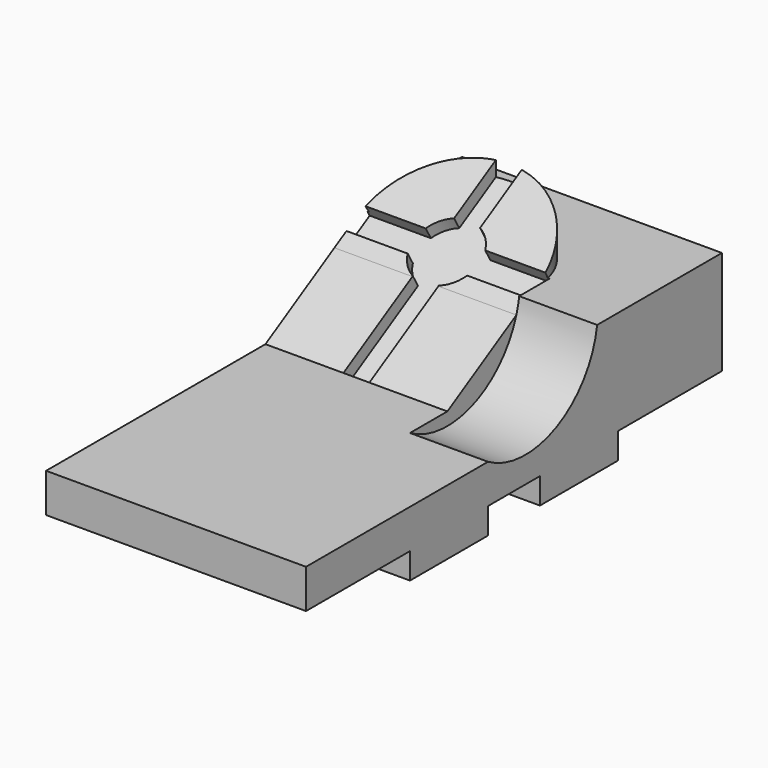
from build123d import *

# Parameters (mm, degrees)
F1_DEPTH  = 30
F0_W      = 37.5
F0_H      = 10
F2_DEPTH  = 100
F4_DEPTH  = 70
F5_W      = 20.9091625453
F5_H      = 25
F6_DEPTH  = 70
F7_DEPTH  = 70
F9_DEPTH  = 5
F12_DEPTH = 17.5


with BuildPart() as f1:
    # F0 (on Right) → F1 (new body)
    with BuildSketch(Plane.YZ):
        with BuildLine():
            Line((-100, 15), (-100, 0))
            Line((-100, 0), (-50, 0))
            Line((-50, 0), (-12.5, 0))
            Line((-12.5, 0), (12.5, 0))
            Line((12.5, 0), (50, 0))
            Line((50, 0), (100, 0))
            Line((100, 0), (100, 40))
            Line((100, 40), (40, 40))
            ThreePointArc((40, 40), (20.4711584909, 13.3855671691), (-12.5, 15))
            Line((-12.5, 15), (-100, 15))
        make_face()
    extrude(amount=-F1_DEPTH)

    # F0 (on Right) → F2 (join)
    with BuildSketch(Plane.YZ):
        with Locations((-31.25, -5)):
            Rectangle(F0_W, F0_H)
        with Locations((31.25, -5)):
            Rectangle(F0_W, F0_H)
    extrude(amount=-F2_DEPTH)

    # F3 (on face) → F4 (join)
    with BuildSketch(Plane(origin=(-30, 0, 0), x_dir=(0, -1, 0), z_dir=(-1, 0, 0))):
        with BuildLine():
            Line((12.5, 15), (-23.473678133, 15))
            ThreePointArc((-23.473678133, 15), (-34.5610974405, 25.633015883), (-40, 40))
            Line((-40, 40), (-100, 40))
            Line((-100, 40), (-100, 0))
            Line((-100, 0), (-50, 0))
            Line((-50, 0), (-12.5, 0))
            Line((-12.5, 0), (12.5, 0))
            Line((12.5, 0), (50, 0))
            Line((50, 0), (100, 0))
            Line((100, 0), (100, 15))
            Line((100, 15), (12.5, 15))
        make_face()
    extrude(amount=F4_DEPTH)

    # F5 (on face) → F6 (join)
    with BuildSketch(Plane(origin=(-100, 0, 0), x_dir=(0, -1, 0), z_dir=(-1, 0, 0))):
        with BuildLine():
            Line((-23.473678133, 15), (-5.478678133, 15))
            Line((-5.478678133, 15), (-38.6573392432, 34.1557089233))
            ThreePointArc((-38.6573392432, 34.1557089233), (-32.7999061901, 23.2030943833), (-23.473678133, 15))
        make_face()
        with Locations((-89.5454187273, 27.5)):
            Rectangle(F5_W, F5_H)
        Polygon((-79.0908374547, 40), (-48.7799483222, 40), (-79.0908374547, 57.5), align=None)
    extrude(amount=-F6_DEPTH)

    # F5 (on face) → F7 (cut)
    with BuildSketch(Plane(origin=(-100, 0, 0), x_dir=(0, -1, 0), z_dir=(-1, 0, 0))):
        with BuildLine():
            Line((-48.7799483222, 40), (-38.6573392432, 34.1557089233))
            ThreePointArc((-38.6573392432, 34.1557089233), (-39.4545948044, 37.048924554), (-40, 40))
            Line((-40, 40), (-48.7799483222, 40))
        make_face()
    extrude(amount=-F7_DEPTH, mode=Mode.SUBTRACT)

    # F8 (on face) → F9 (cut)
    with BuildSketch(Plane(origin=(0, -5.1255209951, 8.8776627788), x_dir=(1, 0, 0), z_dir=(0, -0.5, 0.8660254038))):
        with BuildLine():
            Line((-85.9351158142, 57.2446744423), (-76.4564392374, 57.2446744423))
            ThreePointArc((-76.4564392374, 57.2446744423), (-77.5, 62.2446744423), (-76.4564392374, 67.2446744423))
            Line((-76.4564392374, 67.2446744423), (-85.9351158142, 67.2446744423))
            Line((-85.9351158142, 67.2446744423), (-99.6410161514, 67.2446744423))
            ThreePointArc((-99.6410161514, 67.2446744423), (-99.9101386799, 64.7511096302), (-100, 62.2446744423))
            ThreePointArc((-100, 62.2446744423), (-99.9101386799, 59.7382392545), (-99.6410161514, 57.2446744423))
            Line((-99.6410161514, 57.2446744423), (-85.9351158142, 57.2446744423))
        make_face()
        with BuildLine():
            Line((-60, 73.7011136797), (-60, 96.8856905937))
            ThreePointArc((-60, 96.8856905937), (-62.4935647997, 97.1548131213), (-64.999999975, 97.2446744423))
            ThreePointArc((-64.999999975, 97.2446744423), (-67.5064351754, 97.1548131231), (-70, 96.8856905937))
            Line((-70, 96.8856905937), (-70, 73.7011136797))
            ThreePointArc((-70, 73.7011136797), (-65, 74.7446744423), (-60, 73.7011136797))
        make_face()
        with BuildLine():
            Line((-70, 12.2446744423), (-60, 12.2446744423))
            Line((-60, 12.2446744423), (-60, 50.7882352049))
            ThreePointArc((-60, 50.7882352049), (-65, 49.7446744423), (-70, 50.7882352049))
            Line((-70, 50.7882352049), (-70, 12.2446744423))
        make_face()
        with BuildLine():
            ThreePointArc((-30.3589838486, 57.2446744423), (-30.0898613201, 59.7382392545), (-30, 62.2446744423))
            ThreePointArc((-30, 62.2446744423), (-30.0898613201, 64.7511096302), (-30.3589838486, 67.2446744423))
            Line((-30.3589838486, 67.2446744423), (-53.5435607626, 67.2446744423))
            ThreePointArc((-53.5435607626, 67.2446744423), (-52.7636710884, 64.7985449884), (-52.5, 62.2446744423))
            ThreePointArc((-52.5, 62.2446744423), (-52.7636710884, 59.6908038962), (-53.5435607626, 57.2446744423))
            Line((-53.5435607626, 57.2446744423), (-30.3589838486, 57.2446744423))
        make_face()
        with BuildLine():
            ThreePointArc((-64.999999975, 97.2446744423), (-62.4935647997, 97.1548131213), (-60, 96.8856905937))
            Line((-60, 96.8856905937), (-60, 97.2446744423))
            Line((-60, 97.2446744423), (-64.999999975, 97.2446744423))
        make_face()
        with BuildLine():
            ThreePointArc((-70, 96.8856905937), (-67.5064351754, 97.1548131231), (-64.999999975, 97.2446744423))
            Line((-64.999999975, 97.2446744423), (-70, 97.2446744423))
            Line((-70, 97.2446744423), (-70, 96.8856905937))
        make_face()
        with BuildLine():
            Line((-100, 67.2446744423), (-100, 62.2446744423))
            ThreePointArc((-100, 62.2446744423), (-99.9101386799, 64.7511096302), (-99.6410161514, 67.2446744423))
            Line((-99.6410161514, 67.2446744423), (-100, 67.2446744423))
        make_face()
        with BuildLine():
            Line((-100, 62.2446744423), (-100, 57.2446744423))
            Line((-100, 57.2446744423), (-99.6410161514, 57.2446744423))
            ThreePointArc((-99.6410161514, 57.2446744423), (-99.9101386799, 59.7382392545), (-100, 62.2446744423))
        make_face()
        with BuildLine():
            ThreePointArc((-30.3589838486, 67.2446744423), (-30.0898613201, 64.7511096302), (-30, 62.2446744423))
            Line((-30, 62.2446744423), (-30, 67.2446744423))
            Line((-30, 67.2446744423), (-30.3589838486, 67.2446744423))
        make_face()
        with BuildLine():
            Line((-30.3589838486, 57.2446744423), (-30, 57.2446744423))
            Line((-30, 57.2446744423), (-30, 62.2446744423))
            ThreePointArc((-30, 62.2446744423), (-30.0898613201, 59.7382392545), (-30.3589838486, 57.2446744423))
        make_face()
        with BuildLine():
            ThreePointArc((-70, 50.7882352049), (-65, 49.7446744423), (-60, 50.7882352049))
            ThreePointArc((-60, 50.7882352049), (-56.1611652352, 53.4058396775), (-53.5435607626, 57.2446744423))
            ThreePointArc((-53.5435607626, 57.2446744423), (-52.7636710884, 59.6908038962), (-52.5, 62.2446744423))
            ThreePointArc((-52.5, 62.2446744423), (-52.7636710884, 64.7985449884), (-53.5435607626, 67.2446744423))
            ThreePointArc((-53.5435607626, 67.2446744423), (-56.1611652352, 71.0835092071), (-60, 73.7011136797))
            ThreePointArc((-60, 73.7011136797), (-65, 74.7446744423), (-70, 73.7011136797))
            ThreePointArc((-70, 73.7011136797), (-73.8388347648, 71.0835092071), (-76.4564392374, 67.2446744423))
            ThreePointArc((-76.4564392374, 67.2446744423), (-77.5, 62.2446744423), (-76.4564392374, 57.2446744423))
            ThreePointArc((-76.4564392374, 57.2446744423), (-73.8388347648, 53.4058396775), (-70, 50.7882352049))
        make_face()
    extrude(amount=-F9_DEPTH, mode=Mode.SUBTRACT)

    # F11 (on offset) → F12 (cut)
    with BuildSketch(Plane.XY.offset(57.5)):
        with BuildLine():
            add(Edge.make_bspline(
                [(-65, 79.0908374547), (-100, 79.0908374547), (-100, 48.7799483222)],
                knots=[4.7123889804, 4.7123889804, 4.7123889804, 6.2831853072, 6.2831853072, 6.2831853072], degree=2, weights=[1, 0.7071067812, 1]))
            Line((-65, 79.0908374547), (-100, 79.0908374547))
            Line((-100, 79.0908374547), (-100, 48.7799483222))
        make_face()
        with BuildLine():
            Line((-30, 48.7799483222), (-30, 79.0908374547))
            Line((-30, 79.0908374547), (-65, 79.0908374547))
            add(Edge.make_bspline(
                [(-30, 48.7799483222), (-30, 79.0908374547), (-65, 79.0908374547)],
                knots=[3.1415926536, 3.1415926536, 3.1415926536, 4.7123889804, 4.7123889804, 4.7123889804], degree=2, weights=[1, 0.7071067812, 1]))
        make_face()
    extrude(amount=-F12_DEPTH, mode=Mode.SUBTRACT)


solid = f1.part
